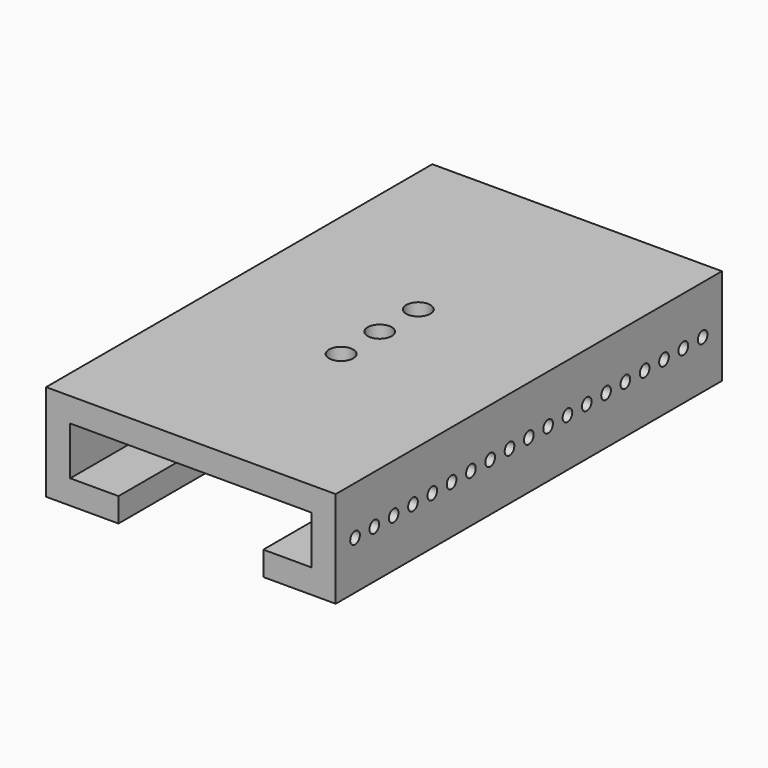
from build123d import *

# Parameters (mm, degrees)
F1_DEPTH = 63.5
F3_R     = 1.5875
F4_DEPTH = 6.35
F2_R     = 3.175
F5_DEPTH = 6.35
F6_DEPTH = 6.35


# Not quite as in the source:
# - a feature names something its author has since deleted; it is built from what else it names


with BuildPart() as f1:
    # F0 (on Front) → F1 (new body, symmetric)
    with BuildSketch(Plane.XZ):
        Polygon((38.1, 3.175), (31.75, 3.175), (-31.75, 3.175), (-38.1, 3.175), (-38.1, -22.225), (-19.05, -22.225), (-19.05, -15.875), (-31.75, -15.875), (-31.75, -3.175), (31.75, -3.175), (31.75, -15.875), (19.05, -15.875), (19.05, -22.225), (38.1, -22.225), align=None)
    extrude(amount=F1_DEPTH, both=True)

    # F3 (on face) → F4 (cut)
    with BuildSketch(Plane.YZ.offset(38.1)):
        with Locations((-57.15, -9.525)):
            Circle(F3_R)
        with Locations((-50.8, -9.525)):
            Circle(F3_R)
        with Locations((-44.45, -9.525)):
            Circle(F3_R)
        with Locations((-38.1, -9.525)):
            Circle(F3_R)
        with Locations((-31.75, -9.525)):
            Circle(F3_R)
        with Locations((-25.4, -9.525)):
            Circle(F3_R)
        with Locations((-19.05, -9.525)):
            Circle(F3_R)
        with Locations((-12.7, -9.525)):
            Circle(F3_R)
        with Locations((-6.35, -9.525)):
            Circle(F3_R)
        with Locations((0, -9.525)):
            Circle(F3_R)
        with Locations((6.35, -9.525)):
            Circle(F3_R)
    extrude(amount=-F4_DEPTH, mode=Mode.SUBTRACT)

    # F2 (on face) → F5 (cut)
    with BuildSketch(Plane.XY.offset(3.175)):
        with Locations((0, 11.2886031434)):
            Circle(F2_R)
        with Locations((0, -1.4113968566)):
            Circle(F2_R)
        with Locations((0, -14.1113968566)):
            Circle(F2_R)
    extrude(amount=-F5_DEPTH, mode=Mode.SUBTRACT)

    # F3 (on face) → F6 (cut)
    with BuildSketch(Plane.YZ.offset(38.1)):
        with Locations((12.7, -9.525)):
            Circle(F3_R)
        with Locations((19.05, -9.525)):
            Circle(F3_R)
        with Locations((25.4, -9.525)):
            Circle(F3_R)
        with Locations((31.75, -9.525)):
            Circle(F3_R)
        with Locations((38.1, -9.525)):
            Circle(F3_R)
        with Locations((44.45, -9.525)):
            Circle(F3_R)
        with Locations((50.8, -9.525)):
            Circle(F3_R)
        with Locations((57.15, -9.525)):
            Circle(F3_R)
    extrude(amount=-F6_DEPTH, mode=Mode.SUBTRACT)


solid = f1.part
